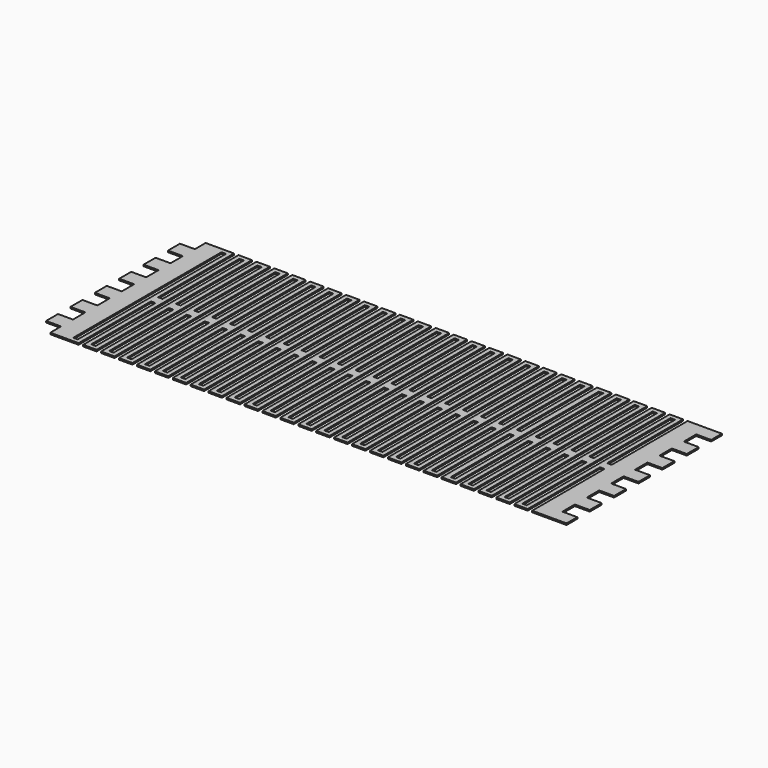
from build123d import *

# Parameters (mm, degrees)
F0_W     = 1.5
F0_H     = 62
F1_DEPTH = 0.5


# Not quite as in the source:
# - ends of sketch curves that miss each other by under 0.0002 mm in the source are joined


with BuildPart() as f1:
    # F0 (on Top) → F1 (new body)
    with BuildSketch(Plane.XY):
        Polygon((-65.4609182477, 0), (-70.4609182477, 0), (-70.4609182477, -4.5), (-75.4609182477, -4.5), (-75.4609182477, -9.5), (-70.4609182477, -9.5), (-70.4609182477, -14.7), (-75.4609182477, -14.7), (-75.4609182477, -19.7), (-70.4609182477, -19.7), (-70.4609182477, -24.9), (-75.4609182477, -24.9), (-75.4609182477, -29.9), (-70.4609182477, -29.9), (-70.4609182477, -35.1), (-75.4609182477, -35.1), (-75.4609182477, -40.1), (-70.4609182477, -40.1), (-70.4609182477, -45.3), (-75.4609182477, -45.3), (-75.4609182477, -50.3), (-70.4609182477, -50.3), (-70.4609182477, -55.5), (-75.4609182477, -55.5), (-75.4609182477, -60.5), (-70.4609182477, -60.5), (-70.4609182477, -65), (-65.4609182477, -65), (-63.9609182477, -65), (-62.4609182477, -65), (-60.9609182477, -65), (-60.9609182477, -34.75), (-59.4609182477, -34.75), (-59.4609182477, -63.5), (-59.4609182477, -65), (-57.9609182477, -65), (-56.4609182477, -65), (-54.9609182477, -65), (-54.9609182477, -34.75), (-53.4609182477, -34.75), (-53.4609182477, -63.5), (-53.4609182477, -65), (-51.9609182477, -65), (-50.4609182477, -65), (-48.9609182477, -65), (-48.9609182477, -63.5), (-48.9609182477, -34.75), (-47.4609182477, -34.75), (-47.4609182477, -63.5), (-47.4609182477, -65), (-45.9609182477, -65), (-44.4609182477, -65), (-42.9609182477, -65), (-42.9609182477, -63.5), (-42.9609182477, -34.75), (-41.4609182477, -34.75), (-41.4609182477, -63.5), (-41.4609182477, -65), (-39.9609182477, -65), (-38.4609182477, -65), (-36.9609182477, -65), (-36.9609182477, -63.5), (-36.9609182477, -34.75), (-35.4609182477, -34.75), (-35.4609182477, -63.5), (-35.4609182477, -65), (-33.9609182477, -65), (-32.4609182477, -65), (-30.9609182477, -65), (-30.9609182477, -63.5), (-30.9609182477, -34.75), (-29.4609182477, -34.75), (-29.4609182477, -63.5), (-29.4609182477, -65), (-27.9609182477, -65), (-26.4609182477, -65), (-24.9609182477, -65), (-24.9609182477, -63.5), (-24.9609182477, -34.75), (-23.4609182477, -34.75), (-23.4609182477, -63.5), (-23.4609182477, -65), (-21.9609182477, -65), (-20.4609182477, -65), (-18.9609182477, -65), (-18.9609182477, -63.5), (-18.9609182477, -34.75), (-17.4609182477, -34.75), (-17.4609182477, -63.5), (-17.4609182477, -65), (-15.9609182477, -65), (-14.4609182477, -65), (-12.9609182477, -65), (-12.9609182477, -63.5), (-12.9609182477, -34.75), (-11.4609182477, -34.75), (-11.4609182477, -63.5), (-11.4609182477, -65), (-9.9609182477, -65), (-8.4609182477, -65), (-6.9609182477, -65), (-6.9609182477, -34.75), (-5.4609182477, -34.75), (-5.4609182477, -63.5), (-5.4609182477, -65), (-3.9609182477, -65), (-2.4609182477, -65), (-0.9609182477, -65), (-0.9609182477, -34.75), (0.5390817523, -34.75), (0.5390817523, -63.5), (0.5390817523, -65), (2.0390817523, -65), (3.5390817523, -65), (5.0390817523, -65), (5.0390817523, -63.5), (5.0390817523, -34.75), (6.5390817523, -34.75), (6.5390817523, -63.4999988079), (6.5390817523, -65), (8.0390817523, -65), (9.5390817523, -65), (11.0390817523, -65), (11.0390817523, -63.5), (11.0390817523, -34.75), (12.5390817523, -34.75), (12.5390817523, -63.4999988079), (12.5390817523, -65), (13.4390817523, -65), (14.0390817523, -65), (15.5390817523, -65), (15.9390817523, -65), (17.0390817523, -65), (17.0390817523, -63.5), (17.0390817523, -34.75), (18.5390817523, -34.75), (18.5390817523, -63.4999988079), (18.5390817523, -65), (20.0390817523, -65), (21.5390817523, -65), (23.0390817523, -65), (23.0390817523, -63.5), (23.0390817523, -34.75), (24.5390817523, -34.75), (24.5390817523, -63.5), (24.5390817523, -65), (26.0390817523, -65), (27.5390817523, -65), (29.0390817523, -65), (29.0390817523, -63.4999976158), (29.0390817523, -34.75), (30.5390817523, -34.75), (30.5390817523, -63.4999988079), (30.5390817523, -65), (32.0390817523, -65), (33.5390817523, -65), (35.0390817523, -65), (35.0390817523, -63.5), (35.0390817523, -34.75), (36.5390817523, -34.75), (36.5390817523, -63.5), (36.5390817523, -65), (38.0390817523, -65), (39.5390817523, -65), (41.0390817523, -65), (41.0390817523, -63.5), (41.0390817523, -34.75), (42.5390817523, -34.75), (42.5390817523, -63.4999988079), (42.5390817523, -65), (44.0390817523, -65), (45.5390817523, -65), (47.0390817523, -65), (47.0390817523, -63.4999976158), (47.0390817523, -34.75), (48.5390817523, -34.75), (48.5390817523, -63.4999976158), (48.5390817523, -65), (50.0390817523, -65), (51.5390817523, -65), (53.0390817523, -65), (53.0390817523, -63.5), (53.0390817523, -34.75), (54.5390817523, -34.75), (54.5390817523, -63.5), (54.5390817523, -65), (56.0390817523, -64.9999976158), (57.5390817523, -65), (59.0390817523, -65), (59.0390817523, -63.4999976158), (59.0390817523, -34.75), (60.5390817523, -34.75), (60.5390817523, -63.4999976158), (60.5390817523, -65), (62.3390817523, -65), (63.8390817523, -65), (65.3390817523, -65), (65.3390817523, -63.5), (65.3390817523, -34.75), (66.8390817523, -34.75), (66.8390817523, -63.5), (66.8390817523, -65), (68.3390817523, -65), (69.8390817523, -65), (71.3390817523, -65), (71.3390817523, -63.5), (71.3390817523, -34.75), (72.8390817523, -34.75), (72.8390817523, -63.5), (72.8390817523, -65), (74.3390817523, -65), (75.8390817523, -65), (77.3390817523, -65), (77.3390817523, -63.5), (77.3390817523, -34.75), (78.8390817523, -34.75), (78.8390817523, -63.5), (78.8390817523, -65), (80.3390817523, -65), (81.8390817523, -65), (83.3390817523, -65), (83.3390817523, -63.5), (83.3390817523, -34.75), (84.8390817523, -34.75), (84.8390817523, -63.5), (84.8390817523, -65), (86.3390817523, -65), (87.8390817523, -65), (89.3390817523, -65), (89.3390817523, -63.5), (89.3390817523, -34.75), (90.8390817523, -34.75), (90.8390817523, -63.5), (90.8390817523, -65), (92.3390817523, -65), (102.3390817523, -65), (102.3390817523, -60.5), (97.3390817523, -60.5), (97.3390817523, -55.3), (102.3390817523, -55.3), (102.3390817523, -50.3), (97.3390817523, -50.3), (97.3390817523, -45.1), (102.3390817523, -45.1), (102.3390817523, -40.1), (97.3390817523, -40.1), (97.3390817523, -34.9), (102.3390817523, -34.9), (102.3390817523, -30.1), (97.3390817523, -30.1), (97.3390817523, -24.9), (102.3390817523, -24.9), (102.3390817523, -19.9), (97.3390817523, -19.9), (97.3390817523, -14.7), (102.3390817523, -14.7), (102.3390817523, -9.7), (97.3390817523, -9.7), (97.3390817523, -4.5), (102.3390817523, -4.5), (102.3390817523, 0), (97.3390817523, 0), (92.3390817523, 0), (90.8390817523, 0), (90.8390817523, -1.5), (90.8390817523, -31.75), (89.3390817523, -31.75), (89.3390817523, -1.5), (89.3390817523, 0), (87.8390817523, 0), (86.3390817523, 0), (84.8390817523, 0), (84.8390817523, -1.5), (84.8390817523, -31.75), (83.3390817523, -31.75), (83.3390817523, -1.5), (83.3390817523, 0), (81.8390817523, 0), (80.3390817523, 0), (78.8390817523, 0), (78.8390817523, -1.5), (78.8390817523, -31.75), (77.3390817523, -31.75), (77.3390817523, -1.5), (77.3390817523, 0), (74.3390817523, 0), (72.8390817523, 0), (72.8390817523, -1.5), (72.8390817523, -31.75), (71.3390817523, -31.75), (71.3390817523, -1.5), (71.3390817523, 0), (69.8390817523, 0), (68.3390817523, 0), (66.8390817523, 0), (66.8390817523, -1.5), (66.8390817523, -31.75), (65.3390817523, -31.75), (65.3390817523, -1.5), (65.3390817523, 0), (63.8390817523, 0), (62.3390817523, 0), (60.5390817523, 0), (60.5390817523, -1.4999976158), (60.5390817523, -31.75), (59.0390817523, -31.75), (59.0390817523, -1.4999976158), (59.0390817523, 0), (57.5390817523, 0), (56.0390817523, 0), (54.5390817523, 0), (54.5390817523, -1.4999976158), (54.5390817523, -2.9999976158), (54.5390817523, -31.75), (53.0390817523, -31.75), (53.0390817523, -2.9999976158), (53.0390817523, -1.4999976158), (53.0390817523, 0), (51.5390817523, 0), (50.0390817523, 0), (48.5390817523, 0), (48.5390817523, -1.4999976158), (48.5390817523, -31.7499992053), (47.0390817523, -31.7499984105), (47.0390817523, -1.4999976158), (47.0390817523, 0), (45.5390817523, 0), (44.0390817523, 0), (42.5390817523, 0), (42.5390817523, -1.5), (42.5390817523, -31.75), (41.0390817523, -31.75), (41.0390817523, -1.5), (41.0390817523, 0), (39.5390817523, 0), (38.0390817523, 0), (36.5390817523, 0), (36.5390817523, -1.5), (36.5390817523, -31.75), (35.0390817523, -31.75), (35.0390817523, -1.5), (35.0390817523, 0), (33.5390817523, 0), (32.0390817523, 0), (30.5390817523, 0), (30.5390817523, -1.5), (30.5390817523, -31.75), (29.0390817523, -31.75), (29.0390817523, -1.5), (29.0390817523, 0), (27.5390817523, 0), (26.0390817523, 0), (24.5390817523, 0), (24.5390817523, -1.5), (24.5390817523, -31.75), (23.0390817523, -31.75), (23.0390817523, -1.5), (23.0390817523, 0), (21.5390817523, 0), (20.0390817523, 0), (18.5390817523, 0), (18.5390817523, -1.5), (18.5390817523, -31.75), (17.0390817523, -31.75), (17.0390817523, -1.5), (17.0390817523, 0), (15.5390817523, 0), (14.0390817523, 0), (13.4390817523, 0), (12.5390817523, 0), (12.5390817523, -1.5), (12.5390817523, -31.75), (11.0390817523, -31.75), (11.0390817523, -1.4999988079), (11.0390817523, 0), (9.5390817523, 0), (8.0390817523, 0), (6.5390817523, 0), (6.5390817523, -1.5), (6.5390817523, -31.75), (5.0390817523, -31.75), (5.0390817523, -1.5), (5.0390817523, 0), (3.5390817523, 0), (2.0390817523, 0), (0.5390817523, 0), (0.5390817523, -1.5), (0.5390817523, -31.75), (-0.9609182477, -31.75), (-0.9609182477, -1.5), (-0.9609182477, 0), (-2.4609182477, 0), (-3.9609182477, 0), (-5.4609182477, 0), (-5.4609182477, -1.5), (-5.4609182477, -31.75), (-6.9609182477, -31.75), (-6.9609182477, -1.5), (-6.9609182477, 0), (-8.4609182477, 0), (-9.9609182477, 0), (-11.4609182477, 0), (-11.4609182477, -1.5), (-11.4609182477, -31.75), (-12.9609182477, -31.75), (-12.9609182477, -1.5), (-12.9609182477, 0), (-14.4609182477, 0), (-15.9609182477, 0), (-17.4609182477, 0), (-17.4609182477, -1.5), (-17.4609182477, -31.75), (-18.9609182477, -31.75), (-18.9609182477, -1.5), (-18.9609182477, 0), (-20.4609182477, 0), (-21.9609182477, 0), (-23.4609182477, 0), (-23.4609182477, -1.5), (-23.4609182477, -31.75), (-24.9609182477, -31.75), (-24.9609182477, -1.5), (-24.9609182477, 0), (-26.4609182477, 0), (-27.9609182477, 0), (-29.4609182477, 0), (-29.4609182477, -1.5), (-29.4609182477, -31.75), (-30.9609182477, -31.75), (-30.9609182477, -1.5), (-30.9609182477, 0), (-32.4609182477, 0), (-33.9609182477, 0), (-35.4609182477, 0), (-35.4609182477, -1.5), (-35.4609182477, -31.75), (-36.9609182477, -31.75), (-36.9609182477, -1.5), (-36.9609182477, 0), (-38.4609182477, 0), (-39.9609182477, 0), (-41.4609182477, 0), (-41.4609182477, -1.5), (-41.4609182477, -31.75), (-42.9609182477, -31.75), (-42.9609182477, -1.5), (-42.9609182477, 0), (-44.4609182477, 0), (-45.9609182477, 0), (-47.4609182477, 0), (-47.4609182477, -1.5), (-47.4609182477, -31.75), (-48.9609182477, -31.75), (-48.9609182477, -1.5), (-48.9609182477, 0), (-50.4609182477, 0), (-51.9609182477, 0), (-53.4609182477, 0), (-53.4609182477, -1.5), (-53.4609182477, -31.75), (-54.9609182477, -31.75), (-54.9609182477, -1.5), (-54.9609182477, 0), (-56.4609182477, 0), (-57.9609182477, 0), (-59.4609182477, 0), (-59.4609182477, -1.5), (-59.4609182477, -31.75), (-60.9609182477, -31.75), (-60.9609182477, -1.5), (-60.9609182477, 0), (-62.4609182477, 0), (-63.9609182477, 0), align=None)
        with Locations((-63.2109182477, -32.5)):
            Rectangle(F0_W, F0_H, mode=Mode.SUBTRACT)
        with Locations((-57.2109182477, -32.5)):
            Rectangle(F0_W, F0_H, mode=Mode.SUBTRACT)
        with Locations((-51.2109182477, -32.5)):
            Rectangle(F0_W, F0_H, mode=Mode.SUBTRACT)
        with Locations((-45.2109182477, -32.5)):
            Rectangle(F0_W, F0_H, mode=Mode.SUBTRACT)
        with Locations((-39.2109182477, -32.5)):
            Rectangle(F0_W, F0_H, mode=Mode.SUBTRACT)
        with Locations((-33.2109182477, -32.5)):
            Rectangle(F0_W, F0_H, mode=Mode.SUBTRACT)
        with Locations((-27.2109182477, -32.5)):
            Rectangle(F0_W, F0_H, mode=Mode.SUBTRACT)
        with Locations((-21.2109182477, -32.5)):
            Rectangle(F0_W, F0_H, mode=Mode.SUBTRACT)
        Polygon((-14.4609182477, -63.5), (-15.9609182477, -63.5), (-15.9609182477, -34.75), (-15.9609182477, -3), (-15.9609182477, -1.5), (-14.4609182477, -1.5), (-14.4609182477, -3), (-14.4609182477, -34.75), align=None, mode=Mode.SUBTRACT)
        with Locations((-9.2109182477, -32.5)):
            Rectangle(F0_W, F0_H, mode=Mode.SUBTRACT)
        with Locations((-3.2109182477, -32.5)):
            Rectangle(F0_W, F0_H, mode=Mode.SUBTRACT)
        with Locations((2.7890817523, -32.4999976158)):
            Rectangle(F0_W, F0_H, mode=Mode.SUBTRACT)
        Polygon((8.0390817523, -31.7499976158), (8.0390817523, -1.4999976158), (9.5390817523, -1.4999976158), (9.5390817523, -31.7499976158), (9.5390817523, -34.75), (9.5390817523, -63.4999976158), (8.0390817523, -63.4999976158), (8.0390817523, -34.75), align=None, mode=Mode.SUBTRACT)
        Polygon((14.0390817523, -31.7499976158), (14.0390817523, -1.4999976158), (15.5390817523, -1.4999976158), (15.5390817523, -31.7499976158), (15.5390817523, -34.75), (15.5390817523, -63.4999976158), (14.0390817523, -63.4999976158), (14.0390817523, -34.75), align=None, mode=Mode.SUBTRACT)
        Polygon((20.0390817523, -34.75), (20.0390817523, -1.4999976158), (21.5390817523, -1.4999976158), (21.5390817523, -34.75), (21.5390817523, -63.4999976158), (20.0390817523, -63.4999976158), align=None, mode=Mode.SUBTRACT)
        Polygon((26.0390817523, -31.7499976158), (26.0390817523, -1.5), (27.5390817523, -1.4999976158), (27.5390817523, -31.7499976158), (27.5390817523, -34.75), (27.5390817523, -63.4999976158), (26.0390817523, -63.4999976158), (26.0390817523, -34.75), align=None, mode=Mode.SUBTRACT)
        Polygon((32.0390817523, -31.75), (32.0390817523, -1.5), (33.5390817523, -1.5), (33.5390817523, -31.75), (33.5390817523, -34.75), (33.5390817523, -63.5), (32.0390817523, -63.5), (32.0390817523, -34.75), align=None, mode=Mode.SUBTRACT)
        Polygon((39.5390817523, -63.5), (38.0390817523, -63.5), (38.0390817523, -34.75), (38.0390817523, -31.7500023842), (38.0390817523, -2.9999976158), (38.0390817523, -1.4999976158), (39.5390817523, -1.4999976158), (39.5390817523, -2.9999976158), (39.5390817523, -31.7500023842), (39.5390817523, -34.75), align=None, mode=Mode.SUBTRACT)
        Polygon((44.0390817523, -31.7499976158), (44.0390817523, -1.4999976158), (45.5390817523, -1.4999976158), (45.5390817523, -31.7499976158), (45.5390817523, -34.75), (45.5390817523, -63.4999976158), (44.0390817523, -63.4999976158), (44.0390817523, -34.75), align=None, mode=Mode.SUBTRACT)
        Polygon((50.0390817523, -31.75), (50.0390817523, -1.5), (51.5390817523, -1.5), (51.5390817523, -31.75), (51.5390817523, -34.75), (51.5390817523, -63.5), (50.0390817523, -63.5), (50.0390817523, -34.75), align=None, mode=Mode.SUBTRACT)
        Polygon((56.0390817523, -31.75), (56.0390817523, -1.5), (57.5390817523, -1.5), (57.5390817523, -31.75), (57.5390817523, -34.75), (57.5390817523, -63.4999976158), (56.0390817523, -63.4999976158), (56.0390817523, -34.75), align=None, mode=Mode.SUBTRACT)
        Polygon((62.3390817523, -31.75), (62.3390817523, -1.5), (63.8390817523, -1.5), (63.8390817523, -31.75), (63.8390817523, -34.75), (63.8390817523, -63.5), (62.3390817523, -63.5), (62.3390817523, -34.75), align=None, mode=Mode.SUBTRACT)
        Polygon((68.3390817523, -31.75), (68.3390817523, -1.5), (69.8390817523, -1.5), (69.8390817523, -31.75), (69.8390817523, -34.75), (69.8390817523, -63.5), (68.3390817523, -63.5), (68.3390817523, -34.75), align=None, mode=Mode.SUBTRACT)
        Polygon((74.3390817523, -1.5), (75.8390817523, -1.5), (75.8390817523, -31.75), (75.8390817523, -34.75), (75.8390817523, -63.5), (74.3390817523, -63.5), (74.3390817523, -34.75), (74.3390817523, -31.75), align=None, mode=Mode.SUBTRACT)
        Polygon((80.3390817523, -1.5), (81.8390817523, -1.5), (81.8390817523, -31.75), (81.8390817523, -34.75), (81.8390817523, -63.5), (80.3390817523, -63.5), (80.3390817523, -34.75), (80.3390817523, -31.75), align=None, mode=Mode.SUBTRACT)
        Polygon((86.3390817523, -1.5), (87.8390817523, -1.5), (87.8390817523, -31.75), (87.8390817523, -34.75), (87.8390817523, -63.5), (86.3390817523, -63.5), (86.3390817523, -34.75), (86.3390817523, -31.75), align=None, mode=Mode.SUBTRACT)
    extrude(amount=F1_DEPTH)


solid = f1.part
